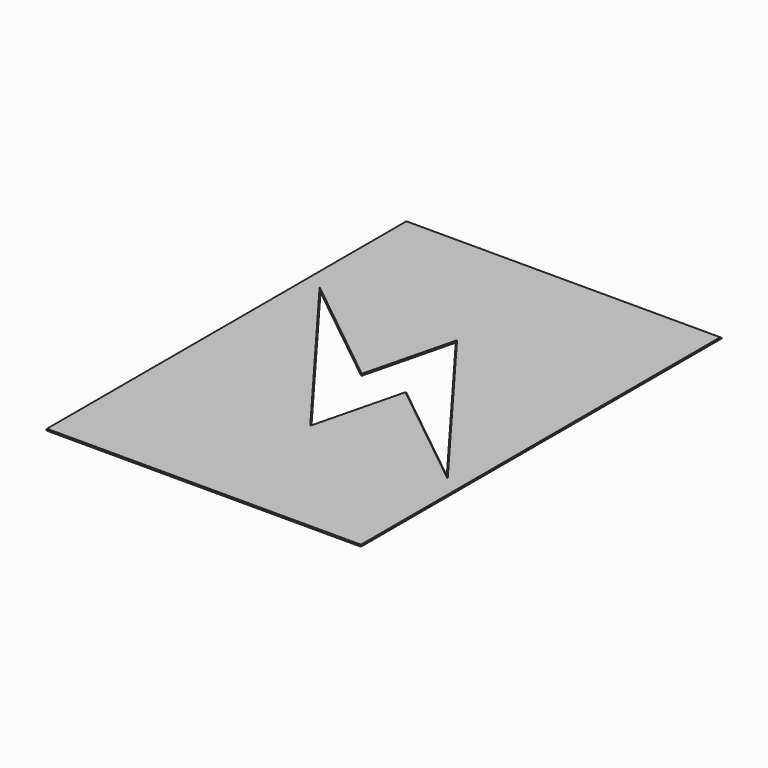
from build123d import *

# Parameters (mm, degrees)
F0_W     = 350
F0_H     = 500
F1_DEPTH = 2
F2_SIZE  = 0.99999


# Not quite as in the source:
# - a fillet or chamfer is up to 0.001 mm smaller than in the source, because OpenCascade refuses the exact size


with BuildPart() as f1:
    # F0 (on Top) → F1 (new body)
    with BuildSketch(Plane.XY):
        Rectangle(F0_W, F0_H)
        Polygon((150, 100), (150, -100), (0, -100), (-150, -100), (-150, 100), (0, 100), align=None, mode=Mode.SUBTRACT)
        Polygon((-150, -100), (0, -100), (-150, 100), align=None)
        Polygon((0, 100), (150, -100), (150, 100), align=None)
        Polygon((-25, 0), (0, 100), (-150, 100), align=None)
        Polygon((0, -100), (150, -100), (25, 0), align=None)
    extrude(amount=F1_DEPTH)

    # F2 (size 1 in the source; OpenCascade refuses exactly that, so slightly less here)
    f2_edges = [f1.edges().sort_by_distance(p)[0] for p in [
        (-75, 0, 2),
        (-87.5, 50, 2),
        (-12.5, 50, 2),
        (75, 0, 2),
        (87.5, -50, 2),
        (12.5, -50, 2),
        (0, -250, 2),
        (175, 0, 2),
        (0, 250, 2),
        (-175, 0, 2),
        (-75, 0, 0),
        (-87.5, 50, 0),
        (-12.5, 50, 0),
        (75, 0, 0),
        (87.5, -50, 0),
        (12.5, -50, 0),
        (0, -250, 0),
        (175, 0, 0),
        (0, 250, 0),
        (-175, 0, 0),
        (-175, -250, 1),
        (175, -250, 1),
        (-175, 250, 1),
    ]]
    chamfer(f2_edges, length=F2_SIZE)


solid = f1.part
